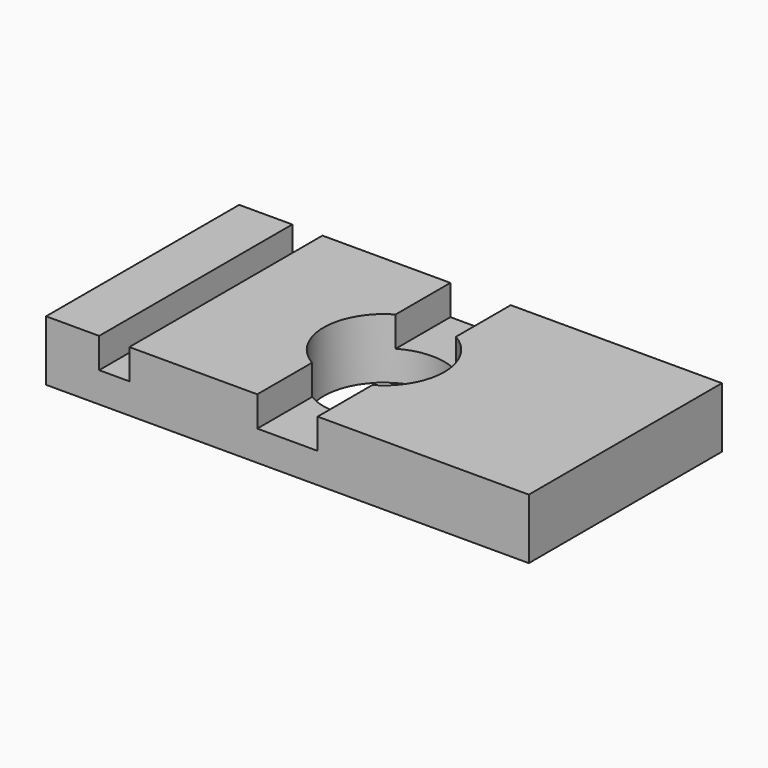
from build123d import *

# Parameters (mm, degrees)
F0_W     = 101.6
F0_H     = 50.8
F0_R     = 12.7
F1_DEPTH = 12.7
F2_W     = 6.35
F2_H     = 50.8
F3_DEPTH = 6.35


with BuildPart() as f1:
    # F0 (on Top) → F1 (new body)
    with BuildSketch(Plane.XY):
        Rectangle(F0_W, F0_H)
        Circle(F0_R, mode=Mode.SUBTRACT)
    extrude(amount=F1_DEPTH)

    # F2 (on face) → F3 (cut)
    with BuildSketch(Plane.XY.offset(12.7)):
        with Locations((-36.4539266646, 0)):
            Rectangle(F2_W, F2_H)
        with BuildLine():
            Line((-6.35, -10.9985226281), (-6.35, -25.4))
            Line((-6.35, -25.4), (6.35, -25.4))
            Line((6.35, -25.4), (6.35, -10.9985226281))
            ThreePointArc((6.35, -10.9985226281), (0, -12.7), (-6.35, -10.9985226281))
        make_face()
        with BuildLine():
            Line((6.35, 25.4), (-6.35, 25.4))
            Line((-6.35, 25.4), (-6.35, 10.9985226281))
            ThreePointArc((-6.35, 10.9985226281), (0, 12.7), (6.35, 10.9985226281))
            Line((6.35, 10.9985226281), (6.35, 25.4))
        make_face()
    extrude(amount=-F3_DEPTH, mode=Mode.SUBTRACT)


solid = f1.part
